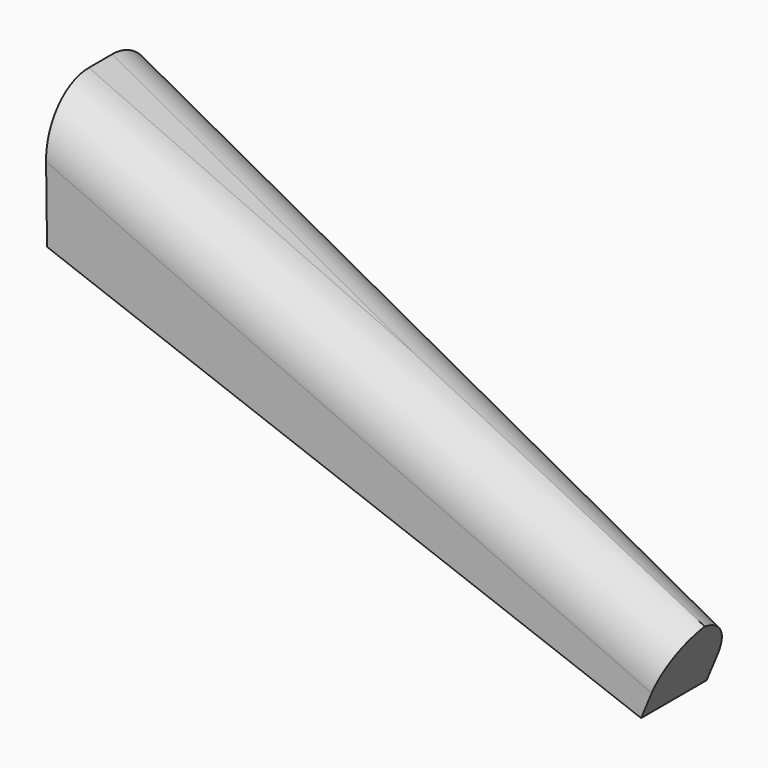
from build123d import *

# Parameters (mm, degrees)
F1_DEPTH     = 25
F2_T1_DEPTH  = 638.9799936737
F3_T1_DEPTH  = 170.2250104198
F3_T3_DEPTH  = 170.2250104198
F3_T8_DEPTH  = 61.8334709535
F3_S9_R      = 10
F3_T10_DEPTH = 33
F3_T14_DEPTH = 61.8334709535
F3_S15_R     = 10
F3_T16_DEPTH = 33


# Not quite as in the source:
# - a fillet or chamfer that OpenCascade refuses, or shapes differently, is made with other operations: its cross-section is extruded or revolved along the edge and cut away or added


with BuildPart() as f1:
    # F0 (on Front) → F1 (new body)
    with BuildSketch(Plane.XZ):
        Polygon((-135, 68.75), (-135, 43.75), (-30, 0), (-24.2307692308, 13.8461538462), align=None)
    extrude(amount=F1_DEPTH)

    # F2: chamfer of 5 x 120 on 2 edges, made by hand

    # F2_s2 → F2_t1 (cut)
    with BuildSketch(Plane(origin=(-124.434022452, 0, -298.6416538849), x_dir=(0, 1, 0), z_dir=(0.3846153846, 0, 0.9230769231))):
        Polygon((-5, 27.6923076923), (0, 147.6923076923), (0, 27.6923076923), align=None)
        Polygon((-20, 27.6923076923), (-25, 147.6923076923), (-25, 27.6923076923), align=None)
    extrude(amount=F2_T1_DEPTH, mode=Mode.SUBTRACT)

    # F3: fillet of radius 10 on 3 edges, made by hand

    # F3_s2 → F3_t1 (cut)
    with BuildSketch(Plane(origin=(-3.3426758621, -0.1551162157, 1.6568297893), x_dir=(0.0463549196, -0.9989250329, 0), z_dir=(-0.8952038609, -0.041541759, 0.443716497))):
        with BuildLine():
            ThreePointArc((8.8845597759, 1.4623687793), (15.8844108663, -1.6017037775), (18.6771013822, -8.7141812364))
            Line((18.6771013822, -8.7141812364), (18.8552852991, 1.2570657903))
            Line((18.8552852991, 1.2570657903), (8.8845597759, 1.4623687793))
        make_face()
    extrude(amount=F3_T1_DEPTH, mode=Mode.SUBTRACT)

    # F3_s4 → F3_t3 (cut)
    with BuildSketch(Plane(origin=(-2.4129672855, 0.1119732721, 1.1960106944), x_dir=(-0.0463549196, -0.9989250329, 0), z_dir=(-0.8952038609, 0.041541759, 0.443716497))):
        with BuildLine():
            ThreePointArc((16.0885660475, 1.976579843), (9.0887149571, -1.0874927139), (6.2960244412, -8.1999701727))
            Line((6.2960244412, -8.1999701727), (6.1178405244, 1.7712768539))
            Line((6.1178405244, 1.7712768539), (16.0885660475, 1.976579843))
        make_face()
    extrude(amount=F3_T3_DEPTH, mode=Mode.SUBTRACT)


with BuildPart() as f3_tool6:
    # F3_s7 → F3_t8 (new body)
    with BuildSketch(Plane.XZ.offset(-18.4167354767)):
        with BuildLine():
            ThreePointArc((-32.6231145704, 18.005901406), (-27.6978305819, 12.5493770531), (-27.8333439195, 5.1999745932))
            Line((-27.8333439195, 5.1999745932), (-24.2307692308, 13.8461538462))
            Line((-24.2307692308, 13.8461538462), (-32.6231145704, 18.005901406))
        make_face()
    extrude(amount=F3_T8_DEPTH)

    # F3_s9 → F3_t10 (cut, symmetric)
    with BuildSketch(Plane(origin=(-27.8408400733, -1.2919487057, 13.7995830572), x_dir=(-0.0463549196, 0.9989250329, 0), z_dir=(0.8952038609, 0.041541759, -0.443716497))):
        with Locations((-8.6786976438, -8.5355120353)):
            Circle(F3_S9_R)
    extrude(amount=F3_T10_DEPTH, both=True, mode=Mode.SUBTRACT)


with BuildPart() as f1_1:
    add(f1.part)

    # F3_t5: cut F3_tool6
    add(f3_tool6.part, mode=Mode.SUBTRACT)


with BuildPart() as f3_tool12:
    # F3_s13 → F3_t14 (new body)
    with BuildSketch(Plane.XZ.offset(-18.4167354767)):
        with BuildLine():
            ThreePointArc((-32.6231145704, 18.005901406), (-27.6978305819, 12.5493770531), (-27.8333439195, 5.1999745932))
            Line((-27.8333439195, 5.1999745932), (-24.2307692308, 13.8461538462))
            Line((-24.2307692308, 13.8461538462), (-32.6231145704, 18.005901406))
        make_face()
    extrude(amount=F3_T14_DEPTH)

    # F3_s15 → F3_t16 (cut, symmetric)
    with BuildSketch(Plane(origin=(-26.9456362125, 1.2504069466, 13.3558665602), x_dir=(0.0463549196, 0.9989250329, 0), z_dir=(0.8952038609, -0.041541759, -0.443716497))):
        with Locations((-16.2944281796, -8.0213009716)):
            Circle(F3_S15_R)
    extrude(amount=F3_T16_DEPTH, both=True, mode=Mode.SUBTRACT)


with BuildPart() as f1_2:
    add(f1_1.part)

    # F3_t11: cut F3_tool12
    add(f3_tool12.part, mode=Mode.SUBTRACT)


solid = f1_2.part
